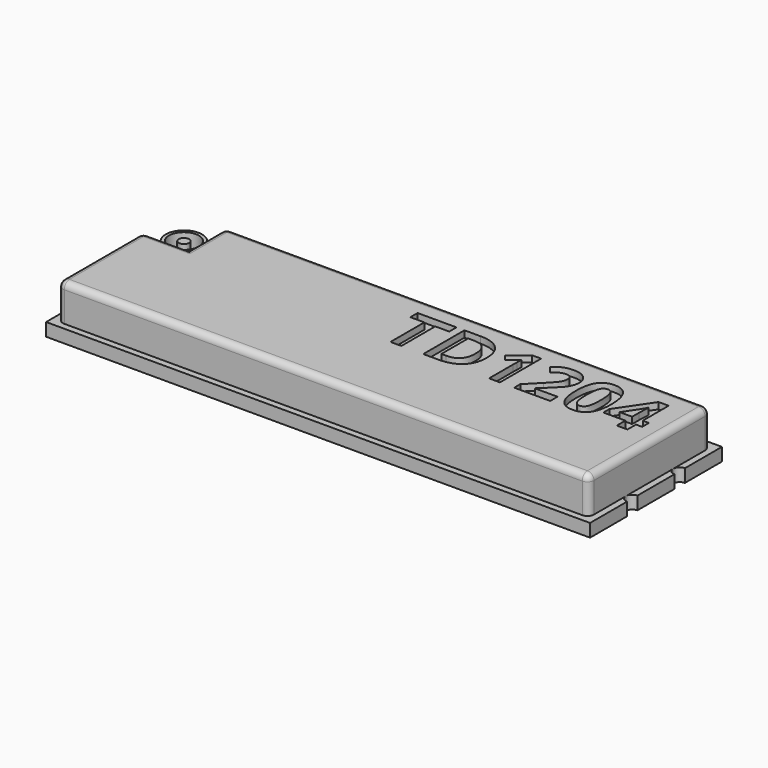
from build123d import *

# Parameters (mm, degrees)
F1_DEPTH     = 2.81
F0_R         = 1.4
F0_R_2       = 1.15
F0_R_3       = 0.4
F2_DEPTH     = 1
F3_DEPTH     = 2
F4_R         = 0.5
F5_TEXT_SIZE = 5.5555555556
F6_DEPTH     = 0.5


# Not quite as in the source:
# - Text() gives the source's letters only with a copy of the font that has no kerning and outlines rounded to 1/6400 em; it was checked with that copy


with BuildPart() as f1:
    # F0 (on Top) → F1 (new body)
    with BuildSketch(Plane.XY):
        Polygon((20.455, -5.85), (20.455, -2.2833333333), (20.455, 2.2833333333), (20.455, 5.85), (16.8883333356, 5.85), (-16.8883333333, 5.85), (-16.8883333333, 2.2833333333), (-20.455, 2.2833333333), (-20.455, -5.85), align=None)
    extrude(amount=F1_DEPTH)

    # F0 (on Top) → F2 (join)
    with BuildSketch(Plane.XY):
        with BuildLine():
            Line((-20.955, 6.35), (-20.955, -6.35))
            Line((-20.955, -6.35), (20.955, -6.35))
            Line((20.955, -6.35), (20.955, -2.7833333333))
            ThreePointArc((20.955, -2.7833333333), (20.6014466094, -2.6368867239), (20.455, -2.2833333333))
            Line((20.455, -2.2833333333), (20.455, -5.85))
            Line((20.455, -5.85), (-20.455, -5.85))
            Line((-20.455, -5.85), (-20.455, 2.2833333333))
            Line((-20.455, 2.2833333333), (-16.8883333333, 2.2833333333))
            Line((-16.8883333333, 2.2833333333), (-16.8883333333, 5.85))
            Line((-16.8883333333, 5.85), (16.8883333356, 5.85))
            ThreePointArc((16.8883333356, 5.85), (16.5347799435, 5.9964466086), (16.3883333333, 6.35))
            Line((16.3883333333, 6.35), (-20.955, 6.35))
        make_face()
        with Locations((-18.6716666667, 4.0666666667)):
            Circle(F0_R, mode=Mode.SUBTRACT)
        with Locations((-18.6716666667, 4.0666666667)):
            Circle(F0_R)
        with Locations((-18.6716666667, 4.0666666667)):
            Circle(F0_R_2, mode=Mode.SUBTRACT)
        with Locations((-18.6716666667, 4.0666666667)):
            Circle(F0_R_2)
        with Locations((-18.6716666667, 4.0666666667)):
            Circle(F0_R_3, mode=Mode.SUBTRACT)
        with BuildLine():
            Line((20.455, 2.2833333333), (20.455, -2.2833333333))
            ThreePointArc((20.455, -2.2833333333), (20.6014466094, -1.9297799427), (20.955, -1.7833333333))
            Line((20.955, -1.7833333333), (20.955, 1.7833333333))
            ThreePointArc((20.955, 1.7833333333), (20.6014466094, 1.9297799427), (20.455, 2.2833333333))
        make_face()
        with BuildLine():
            ThreePointArc((17.3883333333, 6.35), (17.2418867247, 5.9964466102), (16.8883333356, 5.85))
            Line((16.8883333356, 5.85), (20.455, 5.85))
            Line((20.455, 5.85), (20.455, 2.2833333333))
            ThreePointArc((20.455, 2.2833333333), (20.6014466094, 2.6368867239), (20.955, 2.7833333333))
            Line((20.955, 2.7833333333), (20.955, 6.35))
            Line((20.955, 6.35), (17.3883333333, 6.35))
        make_face()
        Polygon((20.455, -5.85), (20.455, -2.2833333333), (20.455, 2.2833333333), (20.455, 5.85), (16.8883333356, 5.85), (-16.8883333333, 5.85), (-16.8883333333, 2.2833333333), (-20.455, 2.2833333333), (-20.455, -5.85), align=None)
        with Locations((-18.6716666667, 4.0666666667)):
            Circle(F0_R_3)
    extrude(amount=-F2_DEPTH)

    # F0 (on Top) → F3 (join)
    with BuildSketch(Plane.XY):
        with Locations((-18.6716666667, 4.0666666667)):
            Circle(F0_R)
        with Locations((-18.6716666667, 4.0666666667)):
            Circle(F0_R_2, mode=Mode.SUBTRACT)
        with Locations((-18.6716666667, 4.0666666667)):
            Circle(F0_R_3)
    extrude(amount=F3_DEPTH)

    # F4
    f4_edges = [f1.edges().sort_by_distance(p)[0] for p in [
        (20.455, 0, 2.81),
        (1.783333, 5.85, 2.81),
        (-16.888333, 4.066667, 2.81),
        (-18.671667, 2.283333, 2.81),
        (-20.455, -1.783333, 2.81),
        (0, -5.85, 2.81),
        (-16.888333, 5.85, 1.405),
        (-20.455, 2.283333, 1.405),
        (-20.455, -5.85, 1.405),
        (20.455, 5.85, 1.405),
        (20.455, -5.85, 1.405),
    ]]
    fillet(f4_edges, radius=F4_R)

    # F5 (on face) → F6 (cut)
    with BuildSketch(Plane.XY.offset(2.81)):
        with Locations((-0.9720833333, 0.35)):
            Text('TD1204', F5_TEXT_SIZE, font='Open Sans', font_style=FontStyle.BOLD, text_align=(TextAlign.LEFT, TextAlign.BOTTOM))
    extrude(amount=-F6_DEPTH, mode=Mode.SUBTRACT)


solid = f1.part
